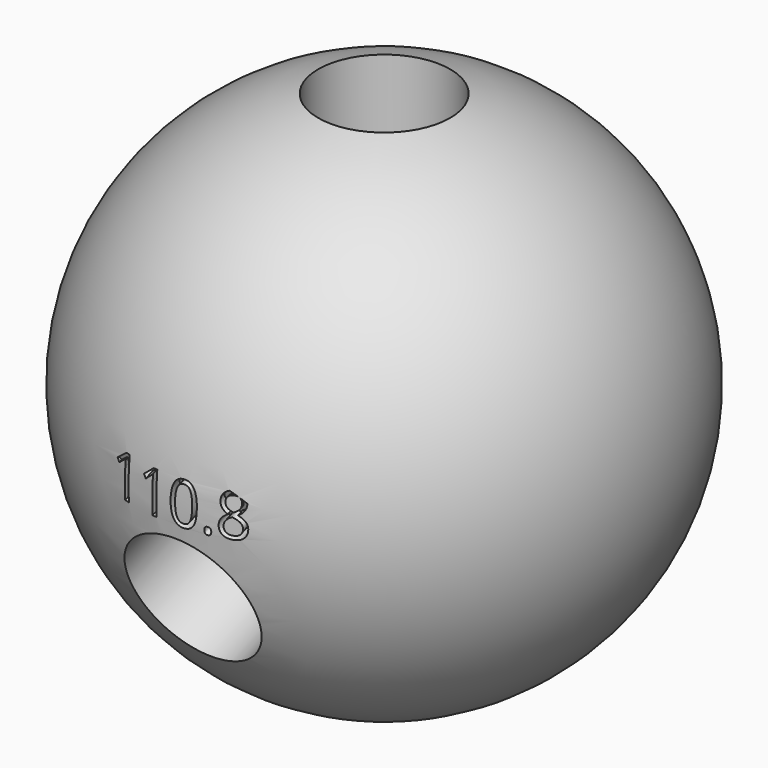
from build123d import *

# Parameters (mm, degrees)
F3_R         = 3.175
F4_DEPTH     = 25.4
F6_ANGLE     = 110.8
F8_TEXT_SIZE = 2.5952509734
F9_DEPTH     = 6.35


# Not quite as in the source:
# - Text() gives the source's letters only with a copy of the font that has no kerning and outlines rounded to 1/6400 em; it was checked with that copy


with BuildPart() as f1:
    # F0 (on Front) → F1 (revolve)
    with BuildSketch(Plane.XZ):
        with BuildLine():
            Line((0, -12.7), (0, 12.7))
            ThreePointArc((0, 12.7), (-12.7, 0), (0, -12.7))
        make_face()
    revolve(axis=Axis((0, 0, 0), (0, 0, -1)))

    # F8 (on offset) → F9 (cut)
    with BuildSketch(Plane(origin=(0, -16.3243933741, -6.2010553311), x_dir=(1, 0, 0), z_dir=(0, -0.9348256764, -0.3551069624))):
        with Locations((-3.2147474121, 3.7727879826)):
            Text('110.8', F8_TEXT_SIZE, font='Open Sans', text_align=(TextAlign.LEFT, TextAlign.BOTTOM))
    extrude(amount=-F9_DEPTH, mode=Mode.SUBTRACT)


with BuildPart() as f4:
    # F3 (on offset) → F4 (new body)
    with BuildSketch(Plane.XY.offset(4.7625)):
        Circle(F3_R)
    extrude(amount=F4_DEPTH)


with BuildPart() as f6_1:
    # F6: copy of F4
    add(f4.part.rotate(Axis((26.6392733902, 0, 0), (1, 0, 0)), F6_ANGLE))


with BuildPart() as f1_1:
    add(f1.part)

    # F10: cut F6_1, F4
    add(f6_1.part, mode=Mode.SUBTRACT)
    add(f4.part, mode=Mode.SUBTRACT)


solid = f1_1.part
